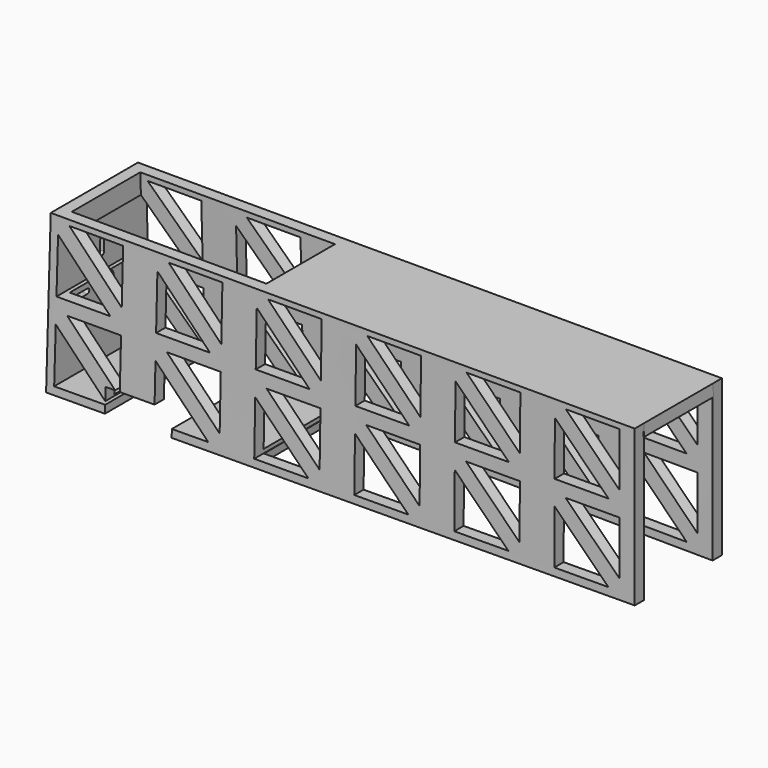
from build123d import *

# Parameters (mm, degrees)
F9_DEPTH       = 3
F9_TAPER       = -3
F3_R           = 2.5
F4_DEPTH       = 3
F8_W           = 97
F8_H           = 22
F5_DEPTH       = 3
F5_TAPER       = -3
F10_DEPTH      = 15.501
F10_DEPTH_BACK = 15.501
F7_W           = 17
F7_H           = 6
F11_DEPTH      = 15.501
F11_DEPTH_BACK = 15.501


with BuildPart() as f2:
    # F0 (on Top) → F2 section 0
    with BuildSketch(Plane.XY):
        Polygon((75, 14), (-75, 15.5), (-75, -15.5), (75, -14), (75, -10.99985), (-22, -11.96985), (-72, -12.46985), (-72, 12.46985), (-22, 11.96985), (75, 10.99985), align=None)
    # F8 (on offset) → F2 section 1
    with BuildSketch(Plane.XY.offset(40)):
        Polygon((-75, -14), (75, -14), (75, -11), (-22, -11), (-72, -11), (-72, 11), (-22, 11), (75, 11), (75, 14), (-75, 14), align=None)
    loft()

    # F0 (on Top) → F9 (join)
    with BuildSketch(Plane.XY):
        Polygon((-22, -11.96985), (-22, 11.96985), (-72, 12.46985), (-72, -12.46985), align=None)
    extrude(amount=F9_DEPTH, taper=F9_TAPER)

    # F3 (on face) → F4 (cut, through all)
    with BuildSketch(Plane(origin=(-75, 0, 0), x_dir=(0, -1, 0), z_dir=(-1, 0, 0))):
        with BuildLine():
            Line((6, 19.375), (9, 19.375))
            ThreePointArc((9, 19.375), (9.625, 20), (9, 20.625))
            Line((9, 20.625), (6, 20.625))
            ThreePointArc((6, 20.625), (5.375, 20), (6, 19.375))
        make_face()
        with Locations((0, 20)):
            Circle(F3_R)
        with BuildLine():
            ThreePointArc((-0.625, 26), (0, 25.375), (0.625, 26))
            Line((0.625, 26), (0.625, 29))
            ThreePointArc((0.625, 29), (0, 29.625), (-0.625, 29))
            Line((-0.625, 29), (-0.625, 26))
        make_face()
        with BuildLine():
            Line((0.625, 11), (0.625, 14))
            ThreePointArc((0.625, 14), (0, 14.625), (-0.625, 14))
            Line((-0.625, 14), (-0.625, 11))
            ThreePointArc((-0.625, 11), (0, 10.375), (0.625, 11))
        make_face()
        with BuildLine():
            ThreePointArc((-9, 20.625), (-9.625, 20), (-9, 19.375))
            Line((-9, 19.375), (-6, 19.375))
            ThreePointArc((-6, 19.375), (-5.375, 20), (-6, 20.625))
            Line((-6, 20.625), (-9, 20.625))
        make_face()
    extrude(amount=-F4_DEPTH, mode=Mode.SUBTRACT)

    # F8 (on offset) → F5 (join)
    with BuildSketch(Plane.XY.offset(40)):
        with Locations((26.5, 0)):
            Rectangle(F8_W, F8_H)
    extrude(amount=-F5_DEPTH, taper=F5_TAPER)

    # F6 (on Front) → F10 (cut, two sides)
    with BuildSketch(Plane.XZ) as f10_sk:
        Polygon((-59.203427, 22), (-73, 35.796573), (-73, 22), align=None)
        Polygon((-56.375, 38.625), (-70.171573, 38.625), (-56.375, 24.828427), align=None)
        Polygon((-56.375, 18.625), (-70.171573, 18.625), (-56.375, 4.828427), align=None)
        Polygon((-59.203427, 2), (-73, 15.796573), (-73, 2), align=None)
        Polygon((-30.875, 38.625), (-44.671573, 38.625), (-30.875, 24.828427), align=None)
        Polygon((-33.703427, 22), (-47.5, 35.796573), (-47.5, 22), align=None)
        Polygon((-30.875, 18.625), (-44.671573, 18.625), (-30.875, 4.828427), align=None)
        Polygon((-33.703427, 2), (-47.5, 15.796573), (-47.5, 2), align=None)
        Polygon((-8.203427, 2), (-22, 15.796573), (-22, 2), align=None)
        Polygon((-5.375, 18.625), (-19.171573, 18.625), (-5.375, 4.828427), align=None)
        Polygon((-8.203427, 22), (-22, 35.796573), (-22, 22), align=None)
        Polygon((-5.375, 38.625), (-19.171573, 38.625), (-5.375, 24.828427), align=None)
        Polygon((17.296573, 22), (3.5, 35.796573), (3.5, 22), align=None)
        Polygon((20.125, 38.625), (6.328427, 38.625), (20.125, 24.828427), align=None)
        Polygon((20.125, 18.625), (6.328427, 18.625), (20.125, 4.828427), align=None)
        Polygon((17.296573, 2), (3.5, 15.796573), (3.5, 2), align=None)
        Polygon((42.796573, 22), (29, 35.796573), (29, 22), align=None)
        Polygon((45.625, 38.625), (31.828427, 38.625), (45.625, 24.828427), align=None)
        Polygon((45.625, 18.625), (31.828427, 18.625), (45.625, 4.828427), align=None)
        Polygon((42.796573, 2), (29, 15.796573), (29, 2), align=None)
        Polygon((68.296573, 2), (54.5, 15.796573), (54.5, 2), align=None)
        Polygon((71.125, 18.625), (57.328427, 18.625), (71.125, 4.828427), align=None)
        Polygon((68.296573, 22), (54.5, 35.796573), (54.5, 22), align=None)
        Polygon((71.125, 38.625), (57.328427, 38.625), (71.125, 24.828427), align=None)
    extrude(amount=F10_DEPTH, mode=Mode.SUBTRACT)
    extrude(f10_sk.sketch, amount=-F10_DEPTH_BACK, mode=Mode.SUBTRACT)

    # F7 (on Front) → F11 (cut, two sides)
    with BuildSketch(Plane.XZ) as f11_sk:
        with Locations((-51.5, 3)):
            Rectangle(F7_W, F7_H)
    extrude(amount=-F11_DEPTH, mode=Mode.SUBTRACT)
    extrude(f11_sk.sketch, amount=F11_DEPTH_BACK, mode=Mode.SUBTRACT)


solid = f2.part
